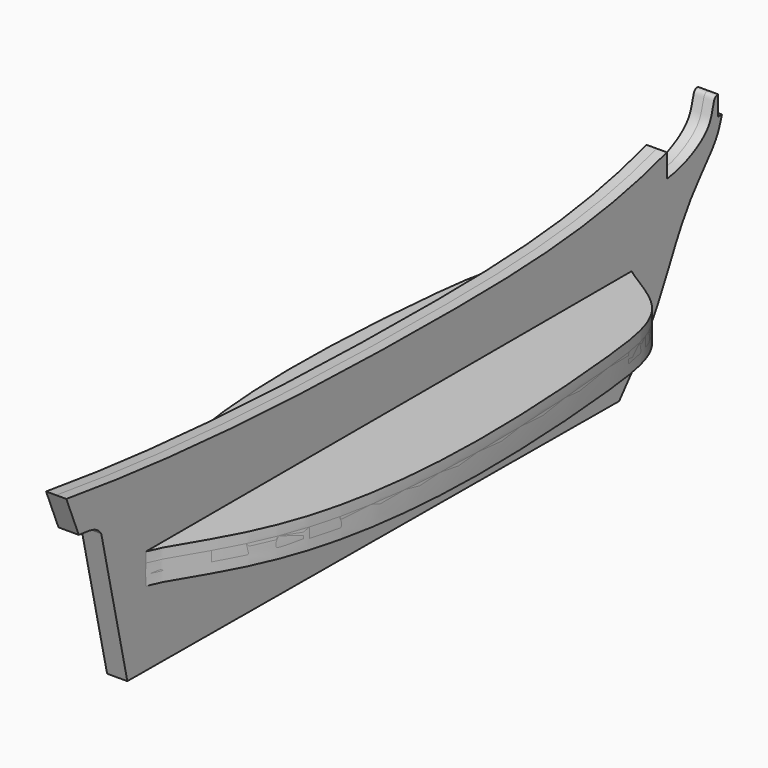
from build123d import *

# Parameters (mm, degrees)
F1_DEPTH = 3
F3_DEPTH = 3
F4_DEPTH = 6


with BuildPart() as f1:
    # F0 (on Right) → F1 (new body, symmetric)
    with BuildSketch(Plane.YZ):
        with BuildLine():
            Line((-157.6520800591, 28.6884028465), (-153.0527025461, 17.4462981522))
            add(Edge.make_bspline(
                [(-153.0527025461, 17.4462981522), (-150.6134849055, 17.2036019536), (-146.5745171917, 16.8017345294), (-145.2322894502, 15.0149770782), (-144.7006613016, 14.3072800711)],
                knots=[0, 0, 0, 0, 0.6039210545, 1, 1, 1, 1], degree=3))
            Line((-144.7006613016, 14.3072800711), (-135.0593864918, -28.0157309026))
            Line((-135.0593864918, -28.0157309026), (47.0432415605, -29.0234107524))
            add(Edge.make_bspline(
                [(47.0432415605, -29.0234107524), (50.647253111, -24.8508082737), (57.7149637062, -16.6680523821), (64.6870070165, -3.4977075876), (72.3742792416, 13.096524661), (83.0860770581, 23.4381483414), (84.5170895995, 28.3117734517), (85.0938931108, 30.276203528)],
                knots=[0, 0, 0, 0, 0.2165605404, 0.424689878, 0.6566012809, 0.8615850098, 1, 1, 1, 1], degree=3))
            Line((85.0938931108, 30.276203528), (83.7138742208, 30.276203528))
            Line((83.7138742208, 30.276203528), (83.7138742208, 36.0895209014))
            add(Edge.make_bspline(
                [(83.7138742208, 36.0895209014), (83.2587014664, 36.0505808822), (81.8080635546, 35.9264788403), (81.632099877, 28.1915858885), (71.325968985, 22.817548486), (66.7259715447, 22.0656692434), (64.7080391645, 21.7358339578)],
                knots=[0, 0, 0, 0, 0.1202197739, 0.3831410383, 0.7293955727, 1, 1, 1, 1], degree=3))
            add(Edge.make_bspline(
                [(64.7080391645, 21.7358339578), (64.7080391645, 24.0533569207), (64.7080391645, 26.3708798836), (64.7080391645, 28.6884028465)],
                knots=[0, 0, 0, 0, 6.9525688887, 6.9525688887, 6.9525688887, 6.9525688887], degree=3))
            add(Edge.make_bspline(
                [(64.7080391645, 28.6884028465), (38.2692925632, 20.3324686736), (-24.4088968897, 18.7009340066), (-110.2832481265, 21.6781254858), (-157.6520800591, 28.6884028465)],
                knots=[0, 0, 0, 0, 0.4448787525, 1, 1, 1, 1], degree=3))
        make_face()
    extrude(amount=F1_DEPTH, both=True)


with BuildPart() as f3:
    # F2 (on Top) → F3 (new body, symmetric)
    with BuildSketch(Plane.XY):
        with BuildLine():
            add(Edge.make_bspline(
                [(0, 54.7371506691), (0.8975022856, 53.5661873997), (3.9748770695, 50.1358264505), (21.722124257, 41.4082381142), (25.9866809631, 14.9070561351), (30.1505980968, -43.8192543552), (23.2688805294, -91.1511136354), (9.7414091497, -116.5857124045), (2.7378078084, -126.8188208342), (1.0830450337, -134.3325078487)],
                knots=[0, 0, 0, 0, 0.0657109202, 0.1817838544, 0.3213945144, 0.5372104353, 0.7320042811, 0.8763200871, 1, 1, 1, 1], degree=3))
            add(Edge.make_bspline(
                [(0, 54.7371506691), (-0.8975022856, 53.5661873997), (-3.9748770695, 50.1358264505), (-21.722124257, 41.4082381142), (-25.9866809631, 14.9070561351), (-30.1505980968, -43.8192543552), (-23.2688805294, -91.1511136354), (-9.7414091497, -116.5857124045), (-2.7378078084, -126.8188208342), (-1.0830450337, -134.3325078487)],
                knots=[0, 0, 0, 0, 0.0657109202, 0.1817838544, 0.3213945144, 0.5372104353, 0.7320042811, 0.8763200871, 1, 1, 1, 1], degree=3))
            Line((-1.0830450337, -134.3325078487), (0, -134.3325078487))
            Line((0, -134.3325078487), (1.0830450337, -134.3325078487))
        make_face()
    extrude(amount=F3_DEPTH, both=True)


with BuildPart() as f4:
    # F2 (on Top) → F4 (new body)
    with BuildSketch(Plane.XY):
        with BuildLine():
            add(Edge.make_bspline(
                [(0, 54.7371506691), (0.8975022856, 53.5661873997), (3.9748770695, 50.1358264505), (21.722124257, 41.4082381142), (25.9866809631, 14.9070561351), (30.1505980968, -43.8192543552), (23.2688805294, -91.1511136354), (9.7414091497, -116.5857124045), (2.7378078084, -126.8188208342), (1.0830450337, -134.3325078487)],
                knots=[0, 0, 0, 0, 0.0657109202, 0.1817838544, 0.3213945144, 0.5372104353, 0.7320042811, 0.8763200871, 1, 1, 1, 1], degree=3))
            add(Edge.make_bspline(
                [(0, 54.7371506691), (-0.8975022856, 53.5661873997), (-3.9748770695, 50.1358264505), (-21.722124257, 41.4082381142), (-25.9866809631, 14.9070561351), (-30.1505980968, -43.8192543552), (-23.2688805294, -91.1511136354), (-9.7414091497, -116.5857124045), (-2.7378078084, -126.8188208342), (-1.0830450337, -134.3325078487)],
                knots=[0, 0, 0, 0, 0.0657109202, 0.1817838544, 0.3213945144, 0.5372104353, 0.7320042811, 0.8763200871, 1, 1, 1, 1], degree=3))
            Line((-1.0830450337, -134.3325078487), (0, -134.3325078487))
            Line((0, -134.3325078487), (1.0830450337, -134.3325078487))
        make_face()
    extrude(amount=-F4_DEPTH)


solid = Compound([f1.part, f3.part, f4.part])
